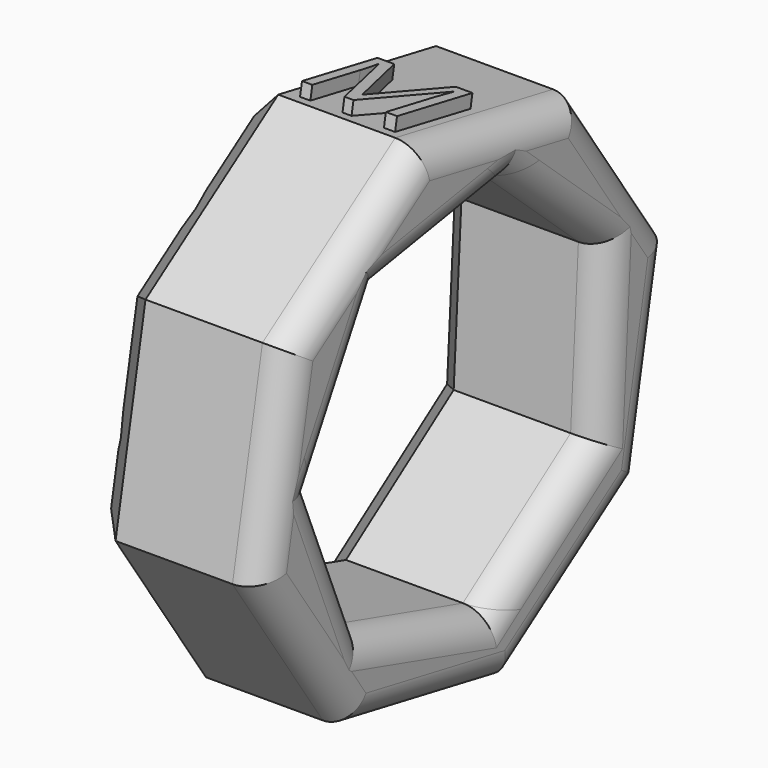
from build123d import *

# Parameters (mm, degrees)
F1_DEPTH      = 30.48
F3_DEPTH      = 60.198
F4_T1_DEPTH   = 60.2839696067
F4_T3_DEPTH   = 60.2839696067
F4_T5_DEPTH   = 60.2839696067
F4_T7_DEPTH   = 60.2839696067
F4_T9_DEPTH   = 60.2839696067
F4_T11_DEPTH  = 60.2839696067
F4_T13_DEPTH  = 60.2839696067
F4_T15_DEPTH  = 60.2839696067
F4_T20_DEPTH  = 54.0223175723
F4_T26_DEPTH  = 54.0223175723
F4_T32_DEPTH  = 54.0223175723
F4_T38_DEPTH  = 54.0223175723
F4_T44_DEPTH  = 54.0223175723
F4_T50_DEPTH  = 54.0223175723
F4_T56_DEPTH  = 54.0223175723
F4_T63_DEPTH  = 54.0223175723
F4_T67_DEPTH  = 54.0223175723
F4_T74_DEPTH  = 54.0223175723
F4_T78_DEPTH  = 54.0223175723
F4_T85_DEPTH  = 54.0223175723
F4_T89_DEPTH  = 54.0223175723
F4_T96_DEPTH  = 54.0223175723
F4_T100_DEPTH = 54.0223175723
F4_T107_DEPTH = 54.0223175723
F4_T111_DEPTH = 54.0223175723
F4_T118_DEPTH = 54.0223175723
F4_T122_DEPTH = 54.0223175723
F4_T129_DEPTH = 54.0223175723
F4_T133_DEPTH = 54.0223175723
F5_T1_DEPTH   = 61.0122687644
F5_T3_DEPTH   = 61.0122687644
F5_T5_DEPTH   = 61.0122687644
F5_T7_DEPTH   = 61.0122687644
F5_T9_DEPTH   = 61.0122687644
F5_T11_DEPTH  = 61.0122687644
F5_T13_DEPTH  = 61.0122687644
F5_T15_DEPTH  = 61.0122687644
F5_T20_DEPTH  = 54.7506167301
F5_T26_DEPTH  = 54.7506167301
F5_T32_DEPTH  = 54.7506167301
F5_T38_DEPTH  = 54.7506167301
F5_T44_DEPTH  = 54.7506167301
F5_T50_DEPTH  = 54.7506167301
F5_T56_DEPTH  = 54.7506167301
F5_T63_DEPTH  = 54.7506167301
F5_T67_DEPTH  = 54.7506167301
F5_T74_DEPTH  = 54.7506167301
F5_T78_DEPTH  = 54.7506167301
F5_T85_DEPTH  = 54.7506167301
F5_T89_DEPTH  = 54.7506167301
F5_T96_DEPTH  = 54.7506167301
F5_T100_DEPTH = 54.7506167301
F5_T107_DEPTH = 54.7506167301
F5_T111_DEPTH = 54.7506167301
F5_T118_DEPTH = 54.7506167301
F5_T122_DEPTH = 54.7506167301
F5_T129_DEPTH = 54.7506167301
F5_T133_DEPTH = 54.7506167301
F6_TEXT_SIZE  = 23.3563218391
F7_DEPTH      = 2.286


# Not quite as in the source:
# - a fillet or chamfer that OpenCascade refuses, or shapes differently, is made with other operations: its cross-section is extruded or revolved along the edge and cut away or added
# - Text() gives the source's letters only with a copy of the font that has no kerning and outlines rounded to 1/6400 em; it was checked with that copy


with BuildPart() as f1:
    # F0 (on Right) → F1 (new body)
    with BuildSketch(Plane.YZ):
        Polygon((9.2812299721, -44.623113081), (38.1161265082, -24.9904852062), (44.623113081, 9.2812299721), (24.9904852062, 38.1161265082), (-9.2812299721, 44.623113081), (-38.1161265082, 24.9904852062), (-44.623113081, -9.2812299721), (-24.9904852062, -38.1161265082), align=None)
    extrude(amount=F1_DEPTH)

    # F2 (on face) → F3 (cut)
    with BuildSketch(Plane(origin=(0, 0, 0), x_dir=(0, -1, 0), z_dir=(-1, 0, 0))):
        Polygon((32.9262018291, 1.9493567982), (19.005082539, 26.9581452719), (-9.227251536, 31.6669005099), (-30.5112770027, 12.5298337769), (-28.8196885698, -16.0424533521), (-5.4262868293, -32.5344459006), (22.0532195697, -24.5273371042), align=None)
    extrude(amount=-F3_DEPTH, mode=Mode.SUBTRACT)

    # F4: fillet of radius 5.08 on 15 edges, made by hand

    # F4_s2 → F4_t1 (cut)
    with BuildSketch(Plane(origin=(0, -29.6129577492, 5.6224533103), x_dir=(1, 0, 0), z_dir=(0, 0.9824488315, -0.1865322853))):
        with BuildLine():
            ThreePointArc((25.4, 42.1086762669), (28.9921024484, 40.6207787153), (30.48, 37.0286762669))
            Line((30.48, 37.0286762669), (30.48, 42.1086762669))
            Line((30.48, 42.1086762669), (25.4, 42.1086762669))
        make_face()
    extrude(amount=F4_T1_DEPTH, mode=Mode.SUBTRACT)

    # F4_s4 → F4_t3 (cut)
    with BuildSketch(Plane(origin=(0, -16.9638483729, 24.9151980981), x_dir=(1, 0, 0), z_dir=(0, 0.562797987, -0.8265944748))):
        with BuildLine():
            ThreePointArc((25.4, 42.1086762669), (28.9921024484, 40.6207787153), (30.48, 37.0286762669))
            Line((30.48, 37.0286762669), (30.48, 42.1086762669))
            Line((30.48, 42.1086762669), (25.4, 42.1086762669))
        make_face()
    extrude(amount=F4_T3_DEPTH, mode=Mode.SUBTRACT)

    # F4_s6 → F4_t5 (cut)
    with BuildSketch(Plane(origin=(0, -24.9151980981, -16.9638483729), x_dir=(1, 0, 0), z_dir=(0, 0.8265944748, 0.562797987))):
        with BuildLine():
            ThreePointArc((25.4, 42.1086762669), (28.9921024484, 40.6207787153), (30.48, 37.0286762669))
            Line((30.48, 37.0286762669), (30.48, 42.1086762669))
            Line((30.48, 42.1086762669), (25.4, 42.1086762669))
        make_face()
    extrude(amount=F4_T5_DEPTH, mode=Mode.SUBTRACT)

    # F4_s8 → F4_t7 (cut)
    with BuildSketch(Plane(origin=(0, 5.6224533103, 29.6129577492), x_dir=(1, 0, 0), z_dir=(0, -0.1865322853, -0.9824488315))):
        with BuildLine():
            ThreePointArc((30.48, 37.0286762669), (28.9921024484, 40.6207787153), (25.4, 42.1086762669))
            Line((25.4, 42.1086762669), (30.48, 42.1086762669))
            Line((30.48, 42.1086762669), (30.48, 37.0286762669))
        make_face()
    extrude(amount=F4_T7_DEPTH, mode=Mode.SUBTRACT)

    # F4_s10 → F4_t9 (cut)
    with BuildSketch(Plane(origin=(0, -5.6224533103, -29.6129577492), x_dir=(1, 0, 0), z_dir=(0, 0.1865322853, 0.9824488315))):
        with BuildLine():
            ThreePointArc((30.48, 37.0286762669), (28.9921024484, 40.6207787153), (25.4, 42.1086762669))
            Line((25.4, 42.1086762669), (30.48, 42.1086762669))
            Line((30.48, 42.1086762669), (30.48, 37.0286762669))
        make_face()
    extrude(amount=F4_T9_DEPTH, mode=Mode.SUBTRACT)

    # F4_s12 → F4_t11 (cut)
    with BuildSketch(Plane(origin=(0, 24.9151980981, 16.9638483729), x_dir=(1, 0, 0), z_dir=(0, -0.8265944748, -0.562797987))):
        with BuildLine():
            ThreePointArc((30.48, 37.0286762669), (28.9921024484, 40.6207787153), (25.4, 42.1086762669))
            Line((25.4, 42.1086762669), (30.48, 42.1086762669))
            Line((30.48, 42.1086762669), (30.48, 37.0286762669))
        make_face()
    extrude(amount=F4_T11_DEPTH, mode=Mode.SUBTRACT)

    # F4_s14 → F4_t13 (cut)
    with BuildSketch(Plane(origin=(0, 16.9638483729, -24.9151980981), x_dir=(1, 0, 0), z_dir=(0, -0.562797987, 0.8265944748))):
        with BuildLine():
            ThreePointArc((30.48, 37.0286762669), (28.9921024484, 40.6207787153), (25.4, 42.1086762669))
            Line((25.4, 42.1086762669), (30.48, 42.1086762669))
            Line((30.48, 42.1086762669), (30.48, 37.0286762669))
        make_face()
    extrude(amount=F4_T13_DEPTH, mode=Mode.SUBTRACT)

    # F4_s16 → F4_t15 (cut)
    with BuildSketch(Plane(origin=(0, 29.6129577492, -5.6224533103), x_dir=(1, 0, 0), z_dir=(0, -0.9824488315, 0.1865322853))):
        with BuildLine():
            ThreePointArc((30.48, 37.0286762669), (28.9921024484, 40.6207787153), (25.4, 42.1086762669))
            Line((25.4, 42.1086762669), (30.48, 42.1086762669))
            Line((30.48, 42.1086762669), (30.48, 37.0286762669))
        make_face()
    extrude(amount=F4_T15_DEPTH, mode=Mode.SUBTRACT)


with BuildPart() as f4_tool18:
    # F4_s19 → F4_t20 (new body)
    with BuildSketch(Plane(origin=(0, 20.0859413302, -18.0598355434), x_dir=(1, 0, 0), z_dir=(0, -0.7436164249, 0.6686064706))):
        with BuildLine():
            ThreePointArc((30.48, 34.7974274292), (28.9921024484, 31.2053249808), (25.4, 29.7174274292))
            Line((25.4, 29.7174274292), (30.48, 29.7174274292))
            Line((30.48, 29.7174274292), (30.48, 34.7974274292))
        make_face()
    extrude(amount=F4_T20_DEPTH)

    split(bisect_by=Plane(origin=(0, -4.8889155015, 29.3125228909), x_dir=(1, 0, 0), z_dir=(0, 0.164513416, -0.9863748456)), keep=Keep.TOP)

    split(bisect_by=Plane(origin=(0, 29.6654827863, -1.7563097876), x_dir=(1, 0, 0), z_dir=(0, -0.9982520478, 0.0591003307)), keep=Keep.TOP)


with BuildPart() as f1_1:
    add(f1.part)

    # F4_t17: cut F4_tool18
    add(f4_tool18.part, mode=Mode.SUBTRACT)


with BuildPart() as f4_tool24:
    # F4_s25 → F4_t26 (new body)
    with BuildSketch(Plane(origin=(0, 26.6431275761, 4.4436980024), x_dir=(1, 0, 0), z_dir=(0, -0.9863748456, -0.164513416))):
        with BuildLine():
            ThreePointArc((30.48, 34.7974274292), (28.9921024484, 31.2053249808), (25.4, 29.7174274292))
            Line((25.4, 29.7174274292), (30.48, 29.7174274292))
            Line((30.48, 29.7174274292), (30.48, 34.7974274292))
        make_face()
    extrude(amount=F4_T26_DEPTH)

    split(bisect_by=Plane(origin=(0, 19.8692642693, 22.0983671434), x_dir=(1, 0, 0), z_dir=(0, -0.6686064706, -0.7436164249)), keep=Keep.TOP)

    split(bisect_by=Plane(origin=(0, -25.965642184, 14.453751035), x_dir=(1, 0, 0), z_dir=(0, 0.8737513449, -0.4863728891)), keep=Keep.TOP)


with BuildPart() as f1_2:
    add(f1_1.part)

    # F4_t23: cut F4_tool24
    add(f4_tool24.part, mode=Mode.SUBTRACT)


with BuildPart() as f4_tool30:
    # F4_s31 → F4_t32 (new body)
    with BuildSketch(Plane(origin=(0, 13.1374953365, 23.6010363174), x_dir=(1, 0, 0), z_dir=(0, -0.4863728891, -0.8737513449))):
        with BuildLine():
            ThreePointArc((30.48, 34.7974274292), (28.9921024484, 31.2053249808), (25.4, 29.7174274292))
            Line((25.4, 29.7174274292), (30.48, 29.7174274292))
            Line((30.48, 29.7174274292), (30.48, 34.7974274292))
        make_face()
    extrude(amount=F4_T32_DEPTH)

    split(bisect_by=Plane(origin=(0, -4.8889155015, 29.3125228909), x_dir=(1, 0, 0), z_dir=(0, 0.164513416, -0.9863748456)), keep=Keep.TOP)

    split(bisect_by=Plane(origin=(0, -27.4897106994, -11.288990153), x_dir=(1, 0, 0), z_dir=(0, 0.9250366898, 0.3798777731)), keep=Keep.TOP)


with BuildPart() as f1_3:
    add(f1_2.part)

    # F4_t29: cut F4_tool30
    add(f4_tool30.part, mode=Mode.SUBTRACT)


with BuildPart() as f4_tool36:
    # F4_s37 → F4_t38 (new body)
    with BuildSketch(Plane(origin=(0, -10.2609388476, 24.986312912), x_dir=(1, 0, 0), z_dir=(0, 0.3798777731, -0.9250366898))):
        with BuildLine():
            ThreePointArc((30.48, 34.7974274292), (28.9921024484, 31.2053249808), (25.4, 29.7174274292))
            Line((25.4, 29.7174274292), (30.48, 29.7174274292))
            Line((30.48, 29.7174274292), (30.48, 34.7974274292))
        make_face()
    extrude(amount=F4_T38_DEPTH)

    split(bisect_by=Plane(origin=(0, -25.965642184, 14.453751035), x_dir=(1, 0, 0), z_dir=(0, 0.8737513449, -0.4863728891)), keep=Keep.TOP)

    split(bisect_by=Plane(origin=(0, -8.3134663702, -28.5308915024), x_dir=(1, 0, 0), z_dir=(0, 0.27975054, 0.960072724)), keep=Keep.TOP)


with BuildPart() as f1_4:
    add(f1_3.part)

    # F4_t35: cut F4_tool36
    add(f4_tool36.part, mode=Mode.SUBTRACT)


with BuildPart() as f4_tool42:
    # F4_s43 → F4_t44 (new body)
    with BuildSketch(Plane(origin=(0, -25.9326767944, 7.556386256), x_dir=(1, 0, 0), z_dir=(0, 0.960072724, -0.27975054))):
        with BuildLine():
            ThreePointArc((30.48, 34.7974274292), (28.9921024484, 31.2053249808), (25.4, 29.7174274292))
            Line((25.4, 29.7174274292), (30.48, 29.7174274292))
            Line((30.48, 29.7174274292), (30.48, 34.7974274292))
        make_face()
    extrude(amount=F4_T44_DEPTH)

    split(bisect_by=Plane(origin=(0, -27.4897106994, -11.288990153), x_dir=(1, 0, 0), z_dir=(0, 0.9250366898, 0.3798777731)), keep=Keep.TOP)

    split(bisect_by=Plane(origin=(0, 17.1229876995, -24.2884496264), x_dir=(1, 0, 0), z_dir=(0, -0.5761934723, 0.8173133319)), keep=Keep.TOP)


with BuildPart() as f1_5:
    add(f1_4.part)

    # F4_t41: cut F4_tool42
    add(f4_tool42.part, mode=Mode.SUBTRACT)


with BuildPart() as f4_tool48:
    # F4_s49 → F4_t50 (new body)
    with BuildSketch(Plane(origin=(0, -22.0765801848, -15.563653373), x_dir=(1, 0, 0), z_dir=(0, 0.8173133319, 0.5761934723))):
        with BuildLine():
            ThreePointArc((30.48, 34.7974274292), (28.9921024484, 31.2053249808), (25.4, 29.7174274292))
            Line((25.4, 29.7174274292), (30.48, 29.7174274292))
            Line((30.48, 29.7174274292), (30.48, 34.7974274292))
        make_face()
    extrude(amount=F4_T50_DEPTH)

    split(bisect_by=Plane(origin=(0, -8.3134663702, -28.5308915024), x_dir=(1, 0, 0), z_dir=(0, 0.27975054, 0.960072724)), keep=Keep.TOP)

    split(bisect_by=Plane(origin=(0, 29.6654827863, -1.7563097876), x_dir=(1, 0, 0), z_dir=(0, -0.9982520478, 0.0591003307)), keep=Keep.TOP)


with BuildPart() as f1_6:
    add(f1_5.part)

    # F4_t47: cut F4_tool48
    add(f4_tool48.part, mode=Mode.SUBTRACT)


with BuildPart() as f4_tool54:
    # F4_s55 → F4_t56 (new body)
    with BuildSketch(Plane(origin=(0, -1.5963684159, -26.9639445715), x_dir=(1, 0, 0), z_dir=(0, 0.0591003307, 0.9982520478))):
        with BuildLine():
            ThreePointArc((30.48, 34.7974274292), (28.9921024484, 31.2053249808), (25.4, 29.7174274292))
            Line((25.4, 29.7174274292), (30.48, 29.7174274292))
            Line((30.48, 29.7174274292), (30.48, 34.7974274292))
        make_face()
    extrude(amount=F4_T56_DEPTH)

    split(bisect_by=Plane(origin=(0, 17.1229876995, -24.2884496264), x_dir=(1, 0, 0), z_dir=(0, -0.5761934723, 0.8173133319)), keep=Keep.TOP)

    split(bisect_by=Plane(origin=(0, 19.8692642693, 22.0983671434), x_dir=(1, 0, 0), z_dir=(0, -0.6686064706, -0.7436164249)), keep=Keep.TOP)


with BuildPart() as f1_7:
    add(f1_6.part)

    # F4_t53: cut F4_tool54
    add(f4_tool54.part, mode=Mode.SUBTRACT)


with BuildPart() as f4_tool61:
    # F4_s62 → F4_t63 (new body)
    with BuildSketch(Plane(origin=(0, 20.0859413302, -18.0598355434), x_dir=(1, 0, 0), z_dir=(0, -0.7436164249, 0.6686064706))):
        with BuildLine():
            ThreePointArc((30.48, 34.7974274292), (28.9921024484, 31.2053249808), (25.4, 29.7174274292))
            Line((25.4, 29.7174274292), (30.48, 29.7174274292))
            Line((30.48, 29.7174274292), (30.48, 34.7974274292))
        make_face()
    extrude(amount=F4_T63_DEPTH)

    split(bisect_by=Plane(origin=(0, 29.6654827863, -1.7563097876), x_dir=(1, 0, 0), z_dir=(0, 0.9982520478, -0.0591003307)), keep=Keep.TOP)


with BuildPart() as f4_tool65:
    # F4_s66 → F4_t67 (new body)
    with BuildSketch(Plane(origin=(0, -1.5963684159, -26.9639445715), x_dir=(1, 0, 0), z_dir=(0, 0.0591003307, 0.9982520478))):
        with BuildLine():
            ThreePointArc((30.48, 34.7974274292), (28.9921024484, 31.2053249808), (25.4, 29.7174274292))
            Line((25.4, 29.7174274292), (30.48, 29.7174274292))
            Line((30.48, 29.7174274292), (30.48, 34.7974274292))
        make_face()
    extrude(amount=F4_T67_DEPTH)

    split(bisect_by=Plane(origin=(0, 19.8692642693, 22.0983671434), x_dir=(1, 0, 0), z_dir=(0, 0.6686064706, 0.7436164249)), keep=Keep.TOP)


with BuildPart() as f4_tool61_1:
    add(f4_tool61.part)

    # F4_t69: intersect F4_tool65
    add(f4_tool65.part, mode=Mode.INTERSECT)


with BuildPart() as f1_8:
    add(f1_7.part)

    # F4_t59: cut F4_tool61
    add(f4_tool61_1.part, mode=Mode.SUBTRACT)


with BuildPart() as f4_tool72:
    # F4_s73 → F4_t74 (new body)
    with BuildSketch(Plane(origin=(0, 20.0859413302, -18.0598355434), x_dir=(1, 0, 0), z_dir=(0, -0.7436164249, 0.6686064706))):
        with BuildLine():
            ThreePointArc((30.48, 34.7974274292), (28.9921024484, 31.2053249808), (25.4, 29.7174274292))
            Line((25.4, 29.7174274292), (30.48, 29.7174274292))
            Line((30.48, 29.7174274292), (30.48, 34.7974274292))
        make_face()
    extrude(amount=F4_T74_DEPTH)

    split(bisect_by=Plane(origin=(0, -4.8889155015, 29.3125228909), x_dir=(1, 0, 0), z_dir=(0, -0.164513416, 0.9863748456)), keep=Keep.TOP)


with BuildPart() as f4_tool76:
    # F4_s77 → F4_t78 (new body)
    with BuildSketch(Plane(origin=(0, 26.6431275761, 4.4436980024), x_dir=(1, 0, 0), z_dir=(0, -0.9863748456, -0.164513416))):
        with BuildLine():
            ThreePointArc((30.48, 34.7974274292), (28.9921024484, 31.2053249808), (25.4, 29.7174274292))
            Line((25.4, 29.7174274292), (30.48, 29.7174274292))
            Line((30.48, 29.7174274292), (30.48, 34.7974274292))
        make_face()
    extrude(amount=F4_T78_DEPTH)

    split(bisect_by=Plane(origin=(0, 19.8692642693, 22.0983671434), x_dir=(1, 0, 0), z_dir=(0, 0.6686064706, 0.7436164249)), keep=Keep.TOP)


with BuildPart() as f4_tool72_1:
    add(f4_tool72.part)

    # F4_t80: intersect F4_tool76
    add(f4_tool76.part, mode=Mode.INTERSECT)


with BuildPart() as f1_9:
    add(f1_8.part)

    # F4_t70: cut F4_tool72
    add(f4_tool72_1.part, mode=Mode.SUBTRACT)


with BuildPart() as f4_tool83:
    # F4_s84 → F4_t85 (new body)
    with BuildSketch(Plane(origin=(0, 26.6431275761, 4.4436980024), x_dir=(1, 0, 0), z_dir=(0, -0.9863748456, -0.164513416))):
        with BuildLine():
            ThreePointArc((30.48, 34.7974274292), (28.9921024484, 31.2053249808), (25.4, 29.7174274292))
            Line((25.4, 29.7174274292), (30.48, 29.7174274292))
            Line((30.48, 29.7174274292), (30.48, 34.7974274292))
        make_face()
    extrude(amount=F4_T85_DEPTH)

    split(bisect_by=Plane(origin=(0, -25.965642184, 14.453751035), x_dir=(1, 0, 0), z_dir=(0, -0.8737513449, 0.4863728891)), keep=Keep.TOP)


with BuildPart() as f4_tool87:
    # F4_s88 → F4_t89 (new body)
    with BuildSketch(Plane(origin=(0, 13.1374953365, 23.6010363174), x_dir=(1, 0, 0), z_dir=(0, -0.4863728891, -0.8737513449))):
        with BuildLine():
            ThreePointArc((30.48, 34.7974274292), (28.9921024484, 31.2053249808), (25.4, 29.7174274292))
            Line((25.4, 29.7174274292), (30.48, 29.7174274292))
            Line((30.48, 29.7174274292), (30.48, 34.7974274292))
        make_face()
    extrude(amount=F4_T89_DEPTH)

    split(bisect_by=Plane(origin=(0, -4.8889155015, 29.3125228909), x_dir=(1, 0, 0), z_dir=(0, -0.164513416, 0.9863748456)), keep=Keep.TOP)


with BuildPart() as f4_tool83_1:
    add(f4_tool83.part)

    # F4_t91: intersect F4_tool87
    add(f4_tool87.part, mode=Mode.INTERSECT)


with BuildPart() as f1_10:
    add(f1_9.part)

    # F4_t81: cut F4_tool83
    add(f4_tool83_1.part, mode=Mode.SUBTRACT)


with BuildPart() as f4_tool94:
    # F4_s95 → F4_t96 (new body)
    with BuildSketch(Plane(origin=(0, 13.1374953365, 23.6010363174), x_dir=(1, 0, 0), z_dir=(0, -0.4863728891, -0.8737513449))):
        with BuildLine():
            ThreePointArc((30.48, 34.7974274292), (28.9921024484, 31.2053249808), (25.4, 29.7174274292))
            Line((25.4, 29.7174274292), (30.48, 29.7174274292))
            Line((30.48, 29.7174274292), (30.48, 34.7974274292))
        make_face()
    extrude(amount=F4_T96_DEPTH)

    split(bisect_by=Plane(origin=(0, -27.4897106994, -11.288990153), x_dir=(1, 0, 0), z_dir=(0, -0.9250366898, -0.3798777731)), keep=Keep.TOP)


with BuildPart() as f4_tool98:
    # F4_s99 → F4_t100 (new body)
    with BuildSketch(Plane(origin=(0, -10.2609388476, 24.986312912), x_dir=(1, 0, 0), z_dir=(0, 0.3798777731, -0.9250366898))):
        with BuildLine():
            ThreePointArc((30.48, 34.7974274292), (28.9921024484, 31.2053249808), (25.4, 29.7174274292))
            Line((25.4, 29.7174274292), (30.48, 29.7174274292))
            Line((30.48, 29.7174274292), (30.48, 34.7974274292))
        make_face()
    extrude(amount=F4_T100_DEPTH)

    split(bisect_by=Plane(origin=(0, -25.965642184, 14.453751035), x_dir=(1, 0, 0), z_dir=(0, -0.8737513449, 0.4863728891)), keep=Keep.TOP)


with BuildPart() as f4_tool94_1:
    add(f4_tool94.part)

    # F4_t102: intersect F4_tool98
    add(f4_tool98.part, mode=Mode.INTERSECT)


with BuildPart() as f1_11:
    add(f1_10.part)

    # F4_t92: cut F4_tool94
    add(f4_tool94_1.part, mode=Mode.SUBTRACT)


with BuildPart() as f4_tool105:
    # F4_s106 → F4_t107 (new body)
    with BuildSketch(Plane(origin=(0, -10.2609388476, 24.986312912), x_dir=(1, 0, 0), z_dir=(0, 0.3798777731, -0.9250366898))):
        with BuildLine():
            ThreePointArc((30.48, 34.7974274292), (28.9921024484, 31.2053249808), (25.4, 29.7174274292))
            Line((25.4, 29.7174274292), (30.48, 29.7174274292))
            Line((30.48, 29.7174274292), (30.48, 34.7974274292))
        make_face()
    extrude(amount=F4_T107_DEPTH)

    split(bisect_by=Plane(origin=(0, -8.3134663702, -28.5308915024), x_dir=(1, 0, 0), z_dir=(0, -0.27975054, -0.960072724)), keep=Keep.TOP)


with BuildPart() as f4_tool109:
    # F4_s110 → F4_t111 (new body)
    with BuildSketch(Plane(origin=(0, -25.9326767944, 7.556386256), x_dir=(1, 0, 0), z_dir=(0, 0.960072724, -0.27975054))):
        with BuildLine():
            ThreePointArc((30.48, 34.7974274292), (28.9921024484, 31.2053249808), (25.4, 29.7174274292))
            Line((25.4, 29.7174274292), (30.48, 29.7174274292))
            Line((30.48, 29.7174274292), (30.48, 34.7974274292))
        make_face()
    extrude(amount=F4_T111_DEPTH)

    split(bisect_by=Plane(origin=(0, -27.4897106994, -11.288990153), x_dir=(1, 0, 0), z_dir=(0, -0.9250366898, -0.3798777731)), keep=Keep.TOP)


with BuildPart() as f4_tool105_1:
    add(f4_tool105.part)

    # F4_t113: intersect F4_tool109
    add(f4_tool109.part, mode=Mode.INTERSECT)


with BuildPart() as f1_12:
    add(f1_11.part)

    # F4_t103: cut F4_tool105
    add(f4_tool105_1.part, mode=Mode.SUBTRACT)


with BuildPart() as f4_tool116:
    # F4_s117 → F4_t118 (new body)
    with BuildSketch(Plane(origin=(0, -25.9326767944, 7.556386256), x_dir=(1, 0, 0), z_dir=(0, 0.960072724, -0.27975054))):
        with BuildLine():
            ThreePointArc((30.48, 34.7974274292), (28.9921024484, 31.2053249808), (25.4, 29.7174274292))
            Line((25.4, 29.7174274292), (30.48, 29.7174274292))
            Line((30.48, 29.7174274292), (30.48, 34.7974274292))
        make_face()
    extrude(amount=F4_T118_DEPTH)

    split(bisect_by=Plane(origin=(0, 17.1229876995, -24.2884496264), x_dir=(1, 0, 0), z_dir=(0, 0.5761934723, -0.8173133319)), keep=Keep.TOP)


with BuildPart() as f4_tool120:
    # F4_s121 → F4_t122 (new body)
    with BuildSketch(Plane(origin=(0, -22.0765801848, -15.563653373), x_dir=(1, 0, 0), z_dir=(0, 0.8173133319, 0.5761934723))):
        with BuildLine():
            ThreePointArc((30.48, 34.7974274292), (28.9921024484, 31.2053249808), (25.4, 29.7174274292))
            Line((25.4, 29.7174274292), (30.48, 29.7174274292))
            Line((30.48, 29.7174274292), (30.48, 34.7974274292))
        make_face()
    extrude(amount=F4_T122_DEPTH)

    split(bisect_by=Plane(origin=(0, -8.3134663702, -28.5308915024), x_dir=(1, 0, 0), z_dir=(0, -0.27975054, -0.960072724)), keep=Keep.TOP)


with BuildPart() as f4_tool116_1:
    add(f4_tool116.part)

    # F4_t124: intersect F4_tool120
    add(f4_tool120.part, mode=Mode.INTERSECT)


with BuildPart() as f1_13:
    add(f1_12.part)

    # F4_t114: cut F4_tool116
    add(f4_tool116_1.part, mode=Mode.SUBTRACT)


with BuildPart() as f4_tool127:
    # F4_s128 → F4_t129 (new body)
    with BuildSketch(Plane(origin=(0, -22.0765801848, -15.563653373), x_dir=(1, 0, 0), z_dir=(0, 0.8173133319, 0.5761934723))):
        with BuildLine():
            ThreePointArc((30.48, 34.7974274292), (28.9921024484, 31.2053249808), (25.4, 29.7174274292))
            Line((25.4, 29.7174274292), (30.48, 29.7174274292))
            Line((30.48, 29.7174274292), (30.48, 34.7974274292))
        make_face()
    extrude(amount=F4_T129_DEPTH)

    split(bisect_by=Plane(origin=(0, 29.6654827863, -1.7563097876), x_dir=(1, 0, 0), z_dir=(0, 0.9982520478, -0.0591003307)), keep=Keep.TOP)


with BuildPart() as f4_tool131:
    # F4_s132 → F4_t133 (new body)
    with BuildSketch(Plane(origin=(0, -1.5963684159, -26.9639445715), x_dir=(1, 0, 0), z_dir=(0, 0.0591003307, 0.9982520478))):
        with BuildLine():
            ThreePointArc((30.48, 34.7974274292), (28.9921024484, 31.2053249808), (25.4, 29.7174274292))
            Line((25.4, 29.7174274292), (30.48, 29.7174274292))
            Line((30.48, 29.7174274292), (30.48, 34.7974274292))
        make_face()
    extrude(amount=F4_T133_DEPTH)

    split(bisect_by=Plane(origin=(0, 17.1229876995, -24.2884496264), x_dir=(1, 0, 0), z_dir=(0, 0.5761934723, -0.8173133319)), keep=Keep.TOP)


with BuildPart() as f4_tool127_1:
    add(f4_tool127.part)

    # F4_t135: intersect F4_tool131
    add(f4_tool131.part, mode=Mode.INTERSECT)


with BuildPart() as f1_14:
    add(f1_13.part)

    # F4_t125: cut F4_tool127
    add(f4_tool127_1.part, mode=Mode.SUBTRACT)

    # F5: chamfer of 5.08 on 15 edges, made by hand

    # F5_s2 → F5_t1 (cut)
    with BuildSketch(Plane(origin=(0, -29.9707160775, 5.6903789634), x_dir=(1, 0, 0), z_dir=(0, 0.9824488315, -0.1865322853))):
        Polygon((5.08, 42.1086762669), (0, 37.0286762669), (0, 42.1086762669), align=None)
    extrude(amount=F5_T1_DEPTH, mode=Mode.SUBTRACT)

    # F5_s4 → F5_t3 (cut)
    with BuildSketch(Plane(origin=(0, -17.1687910229, 25.216202128), x_dir=(1, 0, 0), z_dir=(0, 0.562797987, -0.8265944748))):
        Polygon((5.08, 42.1086762669), (0, 37.0286762669), (0, 42.1086762669), align=None)
    extrude(amount=F5_T3_DEPTH, mode=Mode.SUBTRACT)

    # F5_s6 → F5_t5 (cut)
    with BuildSketch(Plane(origin=(0, -25.216202128, -17.1687910229), x_dir=(1, 0, 0), z_dir=(0, 0.8265944748, 0.562797987))):
        Polygon((5.08, 42.1086762669), (0, 37.0286762669), (0, 42.1086762669), align=None)
    extrude(amount=F5_T5_DEPTH, mode=Mode.SUBTRACT)

    # F5_s8 → F5_t7 (cut)
    with BuildSketch(Plane(origin=(0, 5.6903789634, 29.9707160775), x_dir=(1, 0, 0), z_dir=(0, -0.1865322853, -0.9824488315))):
        Polygon((5.08, 42.1086762669), (0, 37.0286762669), (0, 42.1086762669), align=None)
    extrude(amount=F5_T7_DEPTH, mode=Mode.SUBTRACT)

    # F5_s10 → F5_t9 (cut)
    with BuildSketch(Plane(origin=(0, -5.6903789634, -29.9707160775), x_dir=(1, 0, 0), z_dir=(0, 0.1865322853, 0.9824488315))):
        Polygon((5.08, 42.1086762669), (0, 37.0286762669), (0, 42.1086762669), align=None)
    extrude(amount=F5_T9_DEPTH, mode=Mode.SUBTRACT)

    # F5_s12 → F5_t11 (cut)
    with BuildSketch(Plane(origin=(0, 25.216202128, 17.1687910229), x_dir=(1, 0, 0), z_dir=(0, -0.8265944748, -0.562797987))):
        Polygon((5.08, 42.1086762669), (0, 37.0286762669), (0, 42.1086762669), align=None)
    extrude(amount=F5_T11_DEPTH, mode=Mode.SUBTRACT)

    # F5_s14 → F5_t13 (cut)
    with BuildSketch(Plane(origin=(0, 17.1687910229, -25.216202128), x_dir=(1, 0, 0), z_dir=(0, -0.562797987, 0.8265944748))):
        Polygon((5.08, 42.1086762669), (0, 37.0286762669), (0, 42.1086762669), align=None)
    extrude(amount=F5_T13_DEPTH, mode=Mode.SUBTRACT)

    # F5_s16 → F5_t15 (cut)
    with BuildSketch(Plane(origin=(0, 29.9707160775, -5.6903789634), x_dir=(1, 0, 0), z_dir=(0, -0.9824488315, 0.1865322853))):
        Polygon((5.08, 42.1086762669), (0, 37.0286762669), (0, 42.1086762669), align=None)
    extrude(amount=F5_T15_DEPTH, mode=Mode.SUBTRACT)


with BuildPart() as f5_tool18:
    # F5_s19 → F5_t20 (new body)
    with BuildSketch(Plane(origin=(0, -27.0023155607, -4.5036054935), x_dir=(1, 0, 0), z_dir=(0, 0.9863748456, 0.164513416))):
        Polygon((5.08, -29.7174274292), (0, -34.7974274292), (0, -29.7174274292), align=None)
    extrude(amount=F5_T20_DEPTH)

    split(bisect_by=Plane(origin=(0, -25.965642184, 14.453751035), x_dir=(1, 0, 0), z_dir=(0, 0.8737513449, -0.4863728891)), keep=Keep.TOP)

    split(bisect_by=Plane(origin=(0, 19.8692642693, 22.0983671434), x_dir=(1, 0, 0), z_dir=(0, -0.6686064706, -0.7436164249)), keep=Keep.TOP)


with BuildPart() as f1_15:
    add(f1_14.part)

    # F5_t17: cut F5_tool18
    add(f5_tool18.part, mode=Mode.SUBTRACT)


with BuildPart() as f5_tool24:
    # F5_s25 → F5_t26 (new body)
    with BuildSketch(Plane(origin=(0, -13.3146078192, -23.9192125017), x_dir=(1, 0, 0), z_dir=(0, 0.4863728891, 0.8737513449))):
        Polygon((5.08, -29.7174274292), (0, -34.7974274292), (0, -29.7174274292), align=None)
    extrude(amount=F5_T26_DEPTH)

    split(bisect_by=Plane(origin=(0, -27.4897106994, -11.288990153), x_dir=(1, 0, 0), z_dir=(0, 0.9250366898, 0.3798777731)), keep=Keep.TOP)

    split(bisect_by=Plane(origin=(0, -4.8889155015, 29.3125228909), x_dir=(1, 0, 0), z_dir=(0, 0.164513416, -0.9863748456)), keep=Keep.TOP)


with BuildPart() as f1_16:
    add(f1_15.part)

    # F5_t23: cut F5_tool24
    add(f5_tool24.part, mode=Mode.SUBTRACT)


with BuildPart() as f5_tool30:
    # F5_s31 → F5_t32 (new body)
    with BuildSketch(Plane(origin=(0, 10.3992711787, -25.3231646331), x_dir=(1, 0, 0), z_dir=(0, -0.3798777731, 0.9250366898))):
        Polygon((5.08, -29.7174274292), (0, -34.7974274292), (0, -29.7174274292), align=None)
    extrude(amount=F5_T32_DEPTH)

    split(bisect_by=Plane(origin=(0, -25.965642184, 14.453751035), x_dir=(1, 0, 0), z_dir=(0, 0.8737513449, -0.4863728891)), keep=Keep.TOP)

    split(bisect_by=Plane(origin=(0, -8.3134663702, -28.5308915024), x_dir=(1, 0, 0), z_dir=(0, 0.27975054, 0.960072724)), keep=Keep.TOP)


with BuildPart() as f1_17:
    add(f1_16.part)

    # F5_t29: cut F5_tool30
    add(f5_tool30.part, mode=Mode.SUBTRACT)


with BuildPart() as f5_tool36:
    # F5_s37 → F5_t38 (new body)
    with BuildSketch(Plane(origin=(0, 26.2822868725, -7.6582572973), x_dir=(1, 0, 0), z_dir=(0, -0.960072724, 0.27975054))):
        Polygon((5.08, -29.7174274292), (0, -34.7974274292), (0, -29.7174274292), align=None)
    extrude(amount=F5_T38_DEPTH)

    split(bisect_by=Plane(origin=(0, -27.4897106994, -11.288990153), x_dir=(1, 0, 0), z_dir=(0, 0.9250366898, 0.3798777731)), keep=Keep.TOP)

    split(bisect_by=Plane(origin=(0, 17.1229876995, -24.2884496264), x_dir=(1, 0, 0), z_dir=(0, -0.5761934723, 0.8173133319)), keep=Keep.TOP)


with BuildPart() as f1_18:
    add(f1_17.part)

    # F5_t35: cut F5_tool36
    add(f5_tool36.part, mode=Mode.SUBTRACT)


with BuildPart() as f5_tool42:
    # F5_s43 → F5_t44 (new body)
    with BuildSketch(Plane(origin=(0, 22.3742044904, 15.7734739833), x_dir=(1, 0, 0), z_dir=(0, -0.8173133319, -0.5761934723))):
        Polygon((5.08, -29.7174274292), (0, -34.7974274292), (0, -29.7174274292), align=None)
    extrude(amount=F5_T44_DEPTH)

    split(bisect_by=Plane(origin=(0, -8.3134663702, -28.5308915024), x_dir=(1, 0, 0), z_dir=(0, 0.27975054, 0.960072724)), keep=Keep.TOP)

    split(bisect_by=Plane(origin=(0, 29.6654827863, -1.7563097876), x_dir=(1, 0, 0), z_dir=(0, -0.9982520478, 0.0591003307)), keep=Keep.TOP)


with BuildPart() as f1_19:
    add(f1_18.part)

    # F5_t41: cut F5_tool42
    add(f5_tool42.part, mode=Mode.SUBTRACT)


with BuildPart() as f5_tool48:
    # F5_s49 → F5_t50 (new body)
    with BuildSketch(Plane(origin=(0, 1.6178897764, 27.3274576343), x_dir=(1, 0, 0), z_dir=(0, -0.0591003307, -0.9982520478))):
        Polygon((5.08, -29.7174274292), (0, -34.7974274292), (0, -29.7174274292), align=None)
    extrude(amount=F5_T50_DEPTH)

    split(bisect_by=Plane(origin=(0, 17.1229876995, -24.2884496264), x_dir=(1, 0, 0), z_dir=(0, -0.5761934723, 0.8173133319)), keep=Keep.TOP)

    split(bisect_by=Plane(origin=(0, 19.8692642693, 22.0983671434), x_dir=(1, 0, 0), z_dir=(0, -0.6686064706, -0.7436164249)), keep=Keep.TOP)


with BuildPart() as f1_20:
    add(f1_19.part)

    # F5_t47: cut F5_tool48
    add(f5_tool48.part, mode=Mode.SUBTRACT)


with BuildPart() as f5_tool54:
    # F5_s55 → F5_t56 (new body)
    with BuildSketch(Plane(origin=(0, -20.3567289381, 18.3033083081), x_dir=(1, 0, 0), z_dir=(0, 0.7436164249, -0.6686064706))):
        Polygon((5.08, -29.7174274292), (0, -34.7974274292), (0, -29.7174274292), align=None)
    extrude(amount=F5_T56_DEPTH)

    split(bisect_by=Plane(origin=(0, -4.8889155015, 29.3125228909), x_dir=(1, 0, 0), z_dir=(0, 0.164513416, -0.9863748456)), keep=Keep.TOP)

    split(bisect_by=Plane(origin=(0, 29.6654827863, -1.7563097876), x_dir=(1, 0, 0), z_dir=(0, -0.9982520478, 0.0591003307)), keep=Keep.TOP)


with BuildPart() as f1_21:
    add(f1_20.part)

    # F5_t53: cut F5_tool54
    add(f5_tool54.part, mode=Mode.SUBTRACT)


with BuildPart() as f5_tool61:
    # F5_s62 → F5_t63 (new body)
    with BuildSketch(Plane(origin=(0, -13.3146078192, -23.9192125017), x_dir=(1, 0, 0), z_dir=(0, 0.4863728891, 0.8737513449))):
        Polygon((5.08, -29.7174274292), (0, -34.7974274292), (0, -29.7174274292), align=None)
    extrude(amount=F5_T63_DEPTH)

    split(bisect_by=Plane(origin=(0, -4.8889155015, 29.3125228909), x_dir=(1, 0, 0), z_dir=(0, -0.164513416, 0.9863748456)), keep=Keep.TOP)


with BuildPart() as f5_tool65:
    # F5_s66 → F5_t67 (new body)
    with BuildSketch(Plane(origin=(0, -27.0023155607, -4.5036054935), x_dir=(1, 0, 0), z_dir=(0, 0.9863748456, 0.164513416))):
        Polygon((5.08, -29.7174274292), (0, -34.7974274292), (0, -29.7174274292), align=None)
    extrude(amount=F5_T67_DEPTH)

    split(bisect_by=Plane(origin=(0, -25.965642184, 14.453751035), x_dir=(1, 0, 0), z_dir=(0, -0.8737513449, 0.4863728891)), keep=Keep.TOP)


with BuildPart() as f5_tool61_1:
    add(f5_tool61.part)

    # F5_t69: intersect F5_tool65
    add(f5_tool65.part, mode=Mode.INTERSECT)


with BuildPart() as f1_22:
    add(f1_21.part)

    # F5_t59: cut F5_tool61
    add(f5_tool61_1.part, mode=Mode.SUBTRACT)


with BuildPart() as f5_tool72:
    # F5_s73 → F5_t74 (new body)
    with BuildSketch(Plane(origin=(0, -27.0023155607, -4.5036054935), x_dir=(1, 0, 0), z_dir=(0, 0.9863748456, 0.164513416))):
        Polygon((5.08, -29.7174274292), (0, -34.7974274292), (0, -29.7174274292), align=None)
    extrude(amount=F5_T74_DEPTH)

    split(bisect_by=Plane(origin=(0, 19.8692642693, 22.0983671434), x_dir=(1, 0, 0), z_dir=(0, 0.6686064706, 0.7436164249)), keep=Keep.TOP)


with BuildPart() as f5_tool76:
    # F5_s77 → F5_t78 (new body)
    with BuildSketch(Plane(origin=(0, -20.3567289381, 18.3033083081), x_dir=(1, 0, 0), z_dir=(0, 0.7436164249, -0.6686064706))):
        Polygon((5.08, -29.7174274292), (0, -34.7974274292), (0, -29.7174274292), align=None)
    extrude(amount=F5_T78_DEPTH)

    split(bisect_by=Plane(origin=(0, -4.8889155015, 29.3125228909), x_dir=(1, 0, 0), z_dir=(0, -0.164513416, 0.9863748456)), keep=Keep.TOP)


with BuildPart() as f5_tool72_1:
    add(f5_tool72.part)

    # F5_t80: intersect F5_tool76
    add(f5_tool76.part, mode=Mode.INTERSECT)


with BuildPart() as f1_23:
    add(f1_22.part)

    # F5_t70: cut F5_tool72
    add(f5_tool72_1.part, mode=Mode.SUBTRACT)


with BuildPart() as f5_tool83:
    # F5_s84 → F5_t85 (new body)
    with BuildSketch(Plane(origin=(0, 10.3992711787, -25.3231646331), x_dir=(1, 0, 0), z_dir=(0, -0.3798777731, 0.9250366898))):
        Polygon((5.08, -29.7174274292), (0, -34.7974274292), (0, -29.7174274292), align=None)
    extrude(amount=F5_T85_DEPTH)

    split(bisect_by=Plane(origin=(0, -25.965642184, 14.453751035), x_dir=(1, 0, 0), z_dir=(0, -0.8737513449, 0.4863728891)), keep=Keep.TOP)


with BuildPart() as f5_tool87:
    # F5_s88 → F5_t89 (new body)
    with BuildSketch(Plane(origin=(0, -13.3146078192, -23.9192125017), x_dir=(1, 0, 0), z_dir=(0, 0.4863728891, 0.8737513449))):
        Polygon((5.08, -29.7174274292), (0, -34.7974274292), (0, -29.7174274292), align=None)
    extrude(amount=F5_T89_DEPTH)

    split(bisect_by=Plane(origin=(0, -27.4897106994, -11.288990153), x_dir=(1, 0, 0), z_dir=(0, -0.9250366898, -0.3798777731)), keep=Keep.TOP)


with BuildPart() as f5_tool83_1:
    add(f5_tool83.part)

    # F5_t91: intersect F5_tool87
    add(f5_tool87.part, mode=Mode.INTERSECT)


with BuildPart() as f1_24:
    add(f1_23.part)

    # F5_t81: cut F5_tool83
    add(f5_tool83_1.part, mode=Mode.SUBTRACT)


with BuildPart() as f5_tool94:
    # F5_s95 → F5_t96 (new body)
    with BuildSketch(Plane(origin=(0, 10.3992711787, -25.3231646331), x_dir=(1, 0, 0), z_dir=(0, -0.3798777731, 0.9250366898))):
        Polygon((5.08, -29.7174274292), (0, -34.7974274292), (0, -29.7174274292), align=None)
    extrude(amount=F5_T96_DEPTH)

    split(bisect_by=Plane(origin=(0, -8.3134663702, -28.5308915024), x_dir=(1, 0, 0), z_dir=(0, -0.27975054, -0.960072724)), keep=Keep.TOP)


with BuildPart() as f5_tool98:
    # F5_s99 → F5_t100 (new body)
    with BuildSketch(Plane(origin=(0, 26.2822868725, -7.6582572973), x_dir=(1, 0, 0), z_dir=(0, -0.960072724, 0.27975054))):
        Polygon((5.08, -29.7174274292), (0, -34.7974274292), (0, -29.7174274292), align=None)
    extrude(amount=F5_T100_DEPTH)

    split(bisect_by=Plane(origin=(0, -27.4897106994, -11.288990153), x_dir=(1, 0, 0), z_dir=(0, -0.9250366898, -0.3798777731)), keep=Keep.TOP)


with BuildPart() as f5_tool94_1:
    add(f5_tool94.part)

    # F5_t102: intersect F5_tool98
    add(f5_tool98.part, mode=Mode.INTERSECT)


with BuildPart() as f1_25:
    add(f1_24.part)

    # F5_t92: cut F5_tool94
    add(f5_tool94_1.part, mode=Mode.SUBTRACT)


with BuildPart() as f5_tool105:
    # F5_s106 → F5_t107 (new body)
    with BuildSketch(Plane(origin=(0, 26.2822868725, -7.6582572973), x_dir=(1, 0, 0), z_dir=(0, -0.960072724, 0.27975054))):
        Polygon((5.08, -29.7174274292), (0, -34.7974274292), (0, -29.7174274292), align=None)
    extrude(amount=F5_T107_DEPTH)

    split(bisect_by=Plane(origin=(0, 17.1229876995, -24.2884496264), x_dir=(1, 0, 0), z_dir=(0, 0.5761934723, -0.8173133319)), keep=Keep.TOP)


with BuildPart() as f5_tool109:
    # F5_s110 → F5_t111 (new body)
    with BuildSketch(Plane(origin=(0, 22.3742044904, 15.7734739833), x_dir=(1, 0, 0), z_dir=(0, -0.8173133319, -0.5761934723))):
        Polygon((5.08, -29.7174274292), (0, -34.7974274292), (0, -29.7174274292), align=None)
    extrude(amount=F5_T111_DEPTH)

    split(bisect_by=Plane(origin=(0, -8.3134663702, -28.5308915024), x_dir=(1, 0, 0), z_dir=(0, -0.27975054, -0.960072724)), keep=Keep.TOP)


with BuildPart() as f5_tool105_1:
    add(f5_tool105.part)

    # F5_t113: intersect F5_tool109
    add(f5_tool109.part, mode=Mode.INTERSECT)


with BuildPart() as f1_26:
    add(f1_25.part)

    # F5_t103: cut F5_tool105
    add(f5_tool105_1.part, mode=Mode.SUBTRACT)


with BuildPart() as f5_tool116:
    # F5_s117 → F5_t118 (new body)
    with BuildSketch(Plane(origin=(0, 22.3742044904, 15.7734739833), x_dir=(1, 0, 0), z_dir=(0, -0.8173133319, -0.5761934723))):
        Polygon((5.08, -29.7174274292), (0, -34.7974274292), (0, -29.7174274292), align=None)
    extrude(amount=F5_T118_DEPTH)

    split(bisect_by=Plane(origin=(0, 29.6654827863, -1.7563097876), x_dir=(1, 0, 0), z_dir=(0, 0.9982520478, -0.0591003307)), keep=Keep.TOP)


with BuildPart() as f5_tool120:
    # F5_s121 → F5_t122 (new body)
    with BuildSketch(Plane(origin=(0, 1.6178897764, 27.3274576343), x_dir=(1, 0, 0), z_dir=(0, -0.0591003307, -0.9982520478))):
        Polygon((5.08, -29.7174274292), (0, -34.7974274292), (0, -29.7174274292), align=None)
    extrude(amount=F5_T122_DEPTH)

    split(bisect_by=Plane(origin=(0, 17.1229876995, -24.2884496264), x_dir=(1, 0, 0), z_dir=(0, 0.5761934723, -0.8173133319)), keep=Keep.TOP)


with BuildPart() as f5_tool116_1:
    add(f5_tool116.part)

    # F5_t124: intersect F5_tool120
    add(f5_tool120.part, mode=Mode.INTERSECT)


with BuildPart() as f1_27:
    add(f1_26.part)

    # F5_t114: cut F5_tool116
    add(f5_tool116_1.part, mode=Mode.SUBTRACT)


with BuildPart() as f5_tool127:
    # F5_s128 → F5_t129 (new body)
    with BuildSketch(Plane(origin=(0, -20.3567289381, 18.3033083081), x_dir=(1, 0, 0), z_dir=(0, 0.7436164249, -0.6686064706))):
        Polygon((5.08, -29.7174274292), (0, -34.7974274292), (0, -29.7174274292), align=None)
    extrude(amount=F5_T129_DEPTH)

    split(bisect_by=Plane(origin=(0, 29.6654827863, -1.7563097876), x_dir=(1, 0, 0), z_dir=(0, 0.9982520478, -0.0591003307)), keep=Keep.TOP)


with BuildPart() as f5_tool131:
    # F5_s132 → F5_t133 (new body)
    with BuildSketch(Plane(origin=(0, 1.6178897764, 27.3274576343), x_dir=(1, 0, 0), z_dir=(0, -0.0591003307, -0.9982520478))):
        Polygon((5.08, -29.7174274292), (0, -34.7974274292), (0, -29.7174274292), align=None)
    extrude(amount=F5_T133_DEPTH)

    split(bisect_by=Plane(origin=(0, 19.8692642693, 22.0983671434), x_dir=(1, 0, 0), z_dir=(0, 0.6686064706, 0.7436164249)), keep=Keep.TOP)


with BuildPart() as f5_tool127_1:
    add(f5_tool127.part)

    # F5_t135: intersect F5_tool131
    add(f5_tool131.part, mode=Mode.INTERSECT)


with BuildPart() as f1_28:
    add(f1_27.part)

    # F5_t125: cut F5_tool127
    add(f5_tool127_1.part, mode=Mode.SUBTRACT)

    # F6 (on face) → F7 (join)
    with BuildSketch(Plane(origin=(0, 7.854627617, 41.3696197946), x_dir=(1, 0, 0), z_dir=(0, 0.1865322853, 0.9824488315))):
        with Locations((5.08, -15.5415755512)):
            Text('M', F6_TEXT_SIZE, font='Open Sans', text_align=(TextAlign.LEFT, TextAlign.BOTTOM))
    extrude(amount=F7_DEPTH)


solid = f1_28.part
